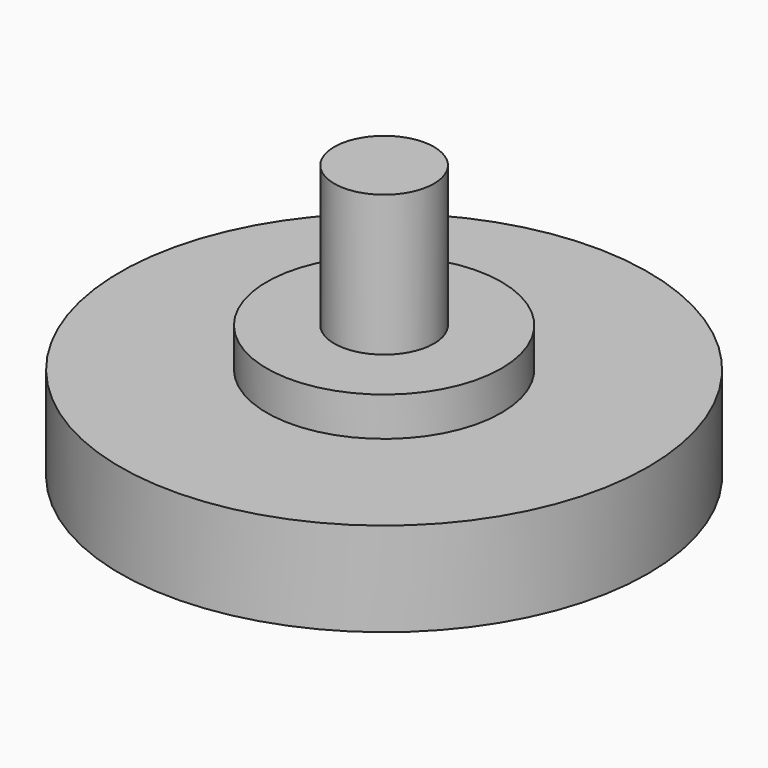
from build123d import *

# Parameters (mm, degrees)
F0_R      = 8.9296875
F0_R_2    = 3.96875
F0_R_3    = 3.175
F0_R_4    = 1.68671875
F1_DEPTH  = 3.175
F2_DEPTH  = 1.3208
F3_DEPTH  = 6.0833
F1_FACE_R = 8.9296875


# Not quite as in the source:
# - a length typed as a fraction of an inch, garbled in the dataset ("3 / 203.2 mm" for 3/8 in), is restored


with BuildPart() as f1:
    # F0 (on Top) → F1 (new body)
    with BuildSketch(Plane.XY):
        Circle(F0_R)
        Circle(F0_R_2, mode=Mode.SUBTRACT)
        Circle(F0_R_2)
        Circle(F0_R_3, mode=Mode.SUBTRACT)
        Circle(F0_R_3)
        Circle(F0_R_4, mode=Mode.SUBTRACT)
        Circle(F0_R_4)
    extrude(amount=-F1_DEPTH)

    # F0 (on Top) → F2 (join)
    with BuildSketch(Plane.XY):
        Circle(F0_R_2)
        Circle(F0_R_3, mode=Mode.SUBTRACT)
        Circle(F0_R_3)
        Circle(F0_R_4, mode=Mode.SUBTRACT)
        Circle(F0_R_4)
    extrude(amount=F2_DEPTH)

    # F0 (on Top) → F3 (join)
    with BuildSketch(Plane.XY):
        Circle(F0_R_4)
    extrude(amount=F3_DEPTH)

    # F1_face (on face) → F4 section 0
    with BuildSketch(Plane(origin=(0, 0, -3.175), x_dir=(1, 0, 0), z_dir=(0, 0, -1)), mode=Mode.PRIVATE) as f4_s0:
        Circle(F1_FACE_R)
    loft([f4_s0.sketch, Vertex(0, 0, 0)], mode=Mode.SUBTRACT)


solid = f1.part
